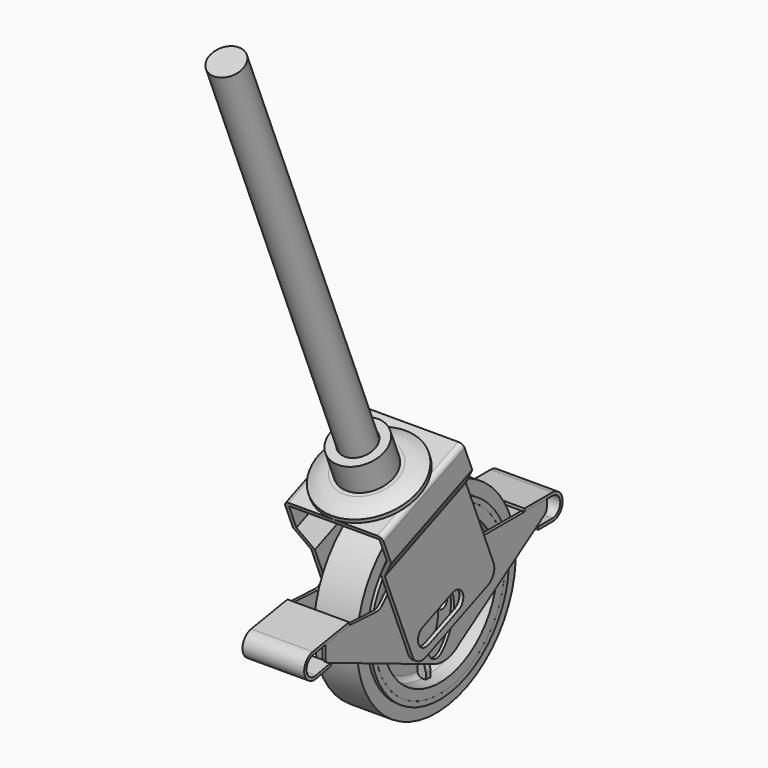
from build123d import *

# Parameters (mm, degrees)
F3_DEPTH  = 3
F4_R      = 5
F5_R      = 6
F6_DEPTH  = 55
F7_COUNT  = 6
F12_R     = 5
F13_DEPTH = 3
F16_DEPTH = 62
F18_DEPTH = 62
F21_DEPTH = 55
F22_R     = 13
F24_DEPTH = 4
F26_R     = 17.5
F27_DEPTH = 4
F30_R     = 17.5
F31_DEPTH = 10
F32_R     = 27
F32_R_2   = 17.5
F33_DEPTH = 30
F35_R     = 17
F36_DEPTH = 500


# Not quite as in the source:
# - ends of sketch curves that miss each other by under 0.0002 mm in the source are joined
# - a pattern or mirror of a feature is missing from the dataset's text; its kind, count and spacing are read off the source's solid


with BuildPart() as f1:
    # F0 (on Front) → F1 (revolve)
    with BuildSketch(Plane.XZ):
        Polygon((0, 82), (0, 0), (27.5, 0), (27.5, 22), (5, 22), (5, 72), (25, 72), (25, 82), align=None)
        Polygon((-27.5, 0), (0, 0), (0, 82), (-25, 82), (-25, 72), (-5, 72), (-5, 22), (-27.5, 22), align=None)
    revolve(axis=Axis((-13.75, 0, 0), (1, 0, 0)))

    # F4
    f4_edges = [f1.edges().sort_by_distance(p)[0] for p in [
        (5, 0, -72),
        (-5, 0, -72),
    ]]
    fillet(f4_edges, radius=F4_R)

    # F5 (on face) → F6 (cut, through all)
    with BuildSketch(Plane.YZ.offset(27.5)):
        Circle(F5_R)
    extrude(amount=-F6_DEPTH, mode=Mode.SUBTRACT)


with BuildPart() as f3:
    # F2 (on Front) → F3 (new body, symmetric)
    with BuildSketch(Plane.XZ):
        with BuildLine():
            ThreePointArc((10, 72), (6.4644660941, 70.5355339059), (5, 67))
            Line((5, 67), (5, 22))
            Line((5, 22), (13.5, 22))
            Line((13.5, 22), (11, 36.5))
            Line((11, 36.5), (11, 56.5))
            Line((11, 56.5), (13.5, 65.5393302441))
            Line((13.5, 65.5393302441), (13.5, 72))
            Line((13.5, 72), (10, 72))
        make_face()
    extrude(amount=F3_DEPTH, both=True)


with BuildPart() as f7_1:
    # F7: instance of F3
    add(f3.part.rotate(Axis((27.5, 0, 0), (1, 0, 0)), 1 * 360 / F7_COUNT))


with BuildPart() as f7_2:
    # F7: instance of F3
    add(f3.part.rotate(Axis((27.5, 0, 0), (1, 0, 0)), 2 * 360 / F7_COUNT))


with BuildPart() as f7_3:
    # F7: instance of F3
    add(f3.part.rotate(Axis((27.5, 0, 0), (1, 0, 0)), 3 * 360 / F7_COUNT))


with BuildPart() as f7_4:
    # F7: instance of F3
    add(f3.part.rotate(Axis((27.5, 0, 0), (1, 0, 0)), 4 * 360 / F7_COUNT))


with BuildPart() as f7_5:
    # F7: instance of F3
    add(f3.part.rotate(Axis((27.5, 0, 0), (1, 0, 0)), 5 * 360 / F7_COUNT))


with BuildPart() as f8_1:
    # F8: instance of F3
    add(f3.part.mirror(Plane.YZ))


with BuildPart() as f8_2:
    # F8: instance of F7_5
    add(f7_5.part.mirror(Plane.YZ))


with BuildPart() as f8_3:
    # F8: instance of F7_4
    add(f7_4.part.mirror(Plane.YZ))


with BuildPart() as f8_4:
    # F8: instance of F7_3
    add(f7_3.part.mirror(Plane.YZ))


with BuildPart() as f8_5:
    # F8: instance of F7_2
    add(f7_2.part.mirror(Plane.YZ))


with BuildPart() as f8_6:
    # F8: instance of F7_1
    add(f7_1.part.mirror(Plane.YZ))


with BuildPart() as f10:
    # F9 (on Top) → F10 (revolve)
    with BuildSketch(Plane.XY):
        Polygon((21.4822281301, -87), (25, -87), (25, -82), (-25, -82), (-25, -87), (-21.5177718699, -87), (-21.5177718699, -100), (21.4822281301, -100), align=None)
    revolve(axis=Axis((27.5, 0, 0), (-1, 0, 0)))


with BuildPart() as f13:
    # F12 (on offset) → F13 (new body)
    with BuildSketch(Plane.YZ.offset(28)):
        with BuildLine():
            Line((127, 41), (31.8588500737, 41))
            ThreePointArc((31.8588500737, 41), (26.284303624, 42.6979260495), (22.6027907005, 47.215113624))
            Line((22.6027907005, 47.215113624), (-3, 109.8275482655))
            Line((-3, 109.8275482655), (-27, 109.8275482655))
            Line((-27, 109.8275482655), (-34.8811647981, 80.414640816))
            ThreePointArc((-34.8811647981, 80.414640816), (-35.8106777129, 78.1251734114), (-37.2731987832, 76.1335189801))
            Line((-37.2731987832, 76.1335189801), (-79.5964464014, 31.3586536425))
            ThreePointArc((-79.5964464014, 31.3586536425), (-83.1487583061, 28.9436013276), (-87.3865234615, 28.2416440355))
            Line((-87.3865234615, 28.2416440355), (-120.9705632925, 30))
            Line((-120.9705632925, 30), (-150.9705632925, 25))
            Line((-150.9705632925, 25), (-150.9705632925, 12.3368176915))
            ThreePointArc((-150.9705632925, 12.3368176915), (-150.1294766363, 9.5613105669), (-147.8891873731, 7.7195802449))
            Line((-147.8891873731, 7.7195802449), (-14.5117444834, -47.7034246791))
            ThreePointArc((-14.5117444834, -47.7034246791), (1.9327525953, -49.5916872083), (16.8755716943, -42.4713517579))
            Line((16.8755716943, -42.4713517579), (124.7486402107, 28.5184114939))
            ThreePointArc((124.7486402107, 28.5184114939), (126.4013180443, 30.3227051329), (127, 32.6951299416))
            Line((127, 32.6951299416), (127, 41))
        make_face()
        with BuildLine():
            ThreePointArc((-9.9237075462, -1.2328943736), (-1.2328943736, 9.9237075462), (9.9237075462, 1.2328943736))
            ThreePointArc((9.9237075462, 1.2328943736), (7.4805498352, -21.4991216683), (-4.8262924538, -40.7671056264))
            ThreePointArc((-4.8262924538, -40.7671056264), (-18.9671056264, -40.5737075462), (-18.7737075462, -26.4328943736))
            ThreePointArc((-18.7737075462, -26.4328943736), (-11.3896021729, -14.8721039988), (-9.9237075462, -1.2328943736))
        make_face(mode=Mode.SUBTRACT)
        with Locations((-53.5, 36.5)):
            Circle(F12_R, mode=Mode.SUBTRACT)
    extrude(amount=F13_DEPTH)


with BuildPart() as f14_1:
    # F14: instance of F13
    add(f13.part.mirror(Plane.YZ))


with BuildPart() as f16:
    # F15 (on face) → F16 (new body, through all)
    with BuildSketch(Plane.YZ.offset(31)):
        with BuildLine():
            ThreePointArc((-163.0315809071, 2.71851264), (-174.8087468604, 10.7370416197), (-166.6145531656, 22.3926683545))
            Line((-166.6145531656, 22.3926683545), (-120.9705632925, 30))
            Line((-120.9705632925, 30), (-121.4637602544, 32.9591817715))
            Line((-121.4637602544, 32.9591817715), (-167.1077501275, 25.351850126))
            ThreePointArc((-167.1077501275, 25.351850126), (-177.7602019307, 10.1995353708), (-162.4498861915, -0.2245523028))
            Line((-162.4498861915, -0.2245523028), (-144.0324838866, 3.4156343068))
            Line((-144.0324838866, 3.4156343068), (-144.6141786022, 6.3586992496))
            Line((-144.6141786022, 6.3586992496), (-163.0315809071, 2.71851264))
        make_face()
    extrude(amount=-F16_DEPTH)


with BuildPart() as f18:
    # F17 (on face) → F18 (new body, through all)
    with BuildSketch(Plane.YZ.offset(31)):
        with BuildLine():
            Line((99, 41), (127, 41))
            Line((127, 41), (134, 41))
            ThreePointArc((134, 41), (143.9999581909, 30.9710832071), (133.942166656, 21.0001672362))
            Line((133.942166656, 21.0001672362), (116.2890405931, 21.0001672362))
            Line((116.2890405931, 21.0001672362), (116.2890405931, 18.0001672362))
            Line((116.2890405931, 18.0001672362), (133.9248166528, 18.0001672362))
            Line((133.9248166528, 18.0001672362), (133.942166656, 18.0001672362))
            ThreePointArc((133.942166656, 18.0001672362), (146.9999678391, 30.9710831706), (134, 44))
            Line((134, 44), (99, 44))
            Line((99, 44), (99, 41))
        make_face()
    extrude(amount=-F18_DEPTH)


with BuildPart() as f21:
    # F20 (on offset) → F21 (new body, symmetric)
    with BuildSketch(Plane(origin=(0, -0.0077183482, -0.0031561024), x_dir=(-1, 0, 0), z_dir=(0, 0.9256059373, 0.3784886376))):
        with BuildLine():
            Line((0, 133.5), (44.5, 133.5))
            ThreePointArc((44.5, 133.5), (45.2071067812, 133.2071067812), (45.5, 132.5))
            Line((45.5, 132.5), (45.5, 108.65))
            Line((45.5, 108.65), (33, 88.65))
            Line((33, 88.65), (33, -17.5))
            Line((33, -17.5), (37, -17.5))
            Line((37, -17.5), (37, 87.5028150944))
            Line((37, 87.5028150944), (49.5, 107.5028150944))
            Line((49.5, 107.5028150944), (49.5, 132.5))
            ThreePointArc((49.5, 132.5), (48.0355339059, 136.0355339059), (44.5, 137.5))
            Line((44.5, 137.5), (0, 137.5))
            Line((0, 137.5), (-44.5, 137.5))
            ThreePointArc((-44.5, 137.5), (-48.0355339059, 136.0355339059), (-49.5, 132.5))
            Line((-49.5, 132.5), (-49.5, 107.5028150944))
            Line((-49.5, 107.5028150944), (-37, 87.5028150944))
            Line((-37, 87.5028150944), (-37, -17.5))
            Line((-37, -17.5), (-33, -17.5))
            Line((-33, -17.5), (-33, 88.65))
            Line((-33, 88.65), (-45.5, 108.65))
            Line((-45.5, 108.65), (-45.5, 132.5))
            ThreePointArc((-45.5, 132.5), (-45.2071067812, 133.2071067812), (-44.5, 133.5))
            Line((-44.5, 133.5), (0, 133.5))
        make_face()
    extrude(amount=F21_DEPTH, both=True)

    # F22
    f22_edges = [f21.edges().sort_by_distance(p)[0] for p in [
        (35, 57.524159, 4.615615),
        (35, -44.292494, -37.018135),
        (-35, -44.292494, -37.018135),
        (-35, 57.524159, 4.615615),
    ]]
    fillet(f22_edges, radius=F22_R)

    # F23 (on face) → F24 (cut, through all)
    with BuildSketch(Plane(origin=(-37, 0, 0), x_dir=(0, -1, 0), z_dir=(-1, 0, 0))):
        with BuildLine():
            Line((-0.8930430629, 11.1687503692), (-0.7934201853, 11.1280140947))
            ThreePointArc((-0.7934201853, 11.1280140947), (-0.8431768183, 11.1485162628), (-0.8930430629, 11.1687503692))
        make_face()
        with BuildLine():
            Line((36.1810606746, -3.9910292413), (-0.7934201853, 11.1280140947))
            Line((-0.7934201853, 11.1280140947), (-0.8930430629, 11.1687503692))
            ThreePointArc((-0.8930430629, 11.1687503692), (-13.9403236987, 5.5367785502), (-8.1813671125, -7.4549518041))
            Line((-8.1813671125, -7.4549518041), (28.6106000979, -22.5028666972))
            ThreePointArc((28.6106000979, -22.5028666972), (41.6521265419, -17.0323326076), (36.1810606746, -3.9910292413))
        make_face()
    f24 = extrude(amount=-F24_DEPTH, mode=Mode.SUBTRACT)

    # F24_copies: F24 across plane
    add(f24.mirror(Plane(origin=(0, 0, 0), x_dir=(0, 0, 1), z_dir=(1, 0, 0))), mode=Mode.SUBTRACT)

    # F26 (on face) → F27 (cut, through all)
    with BuildSketch(Plane(origin=(0, -52.0421876702, 127.2708163818), x_dir=(1, 0, 0), z_dir=(0, -0.3784886376, 0.9256059373))):
        with Locations((0, -5.0083386979)):
            Circle(F26_R)
    extrude(amount=-F27_DEPTH, mode=Mode.SUBTRACT)


with BuildPart() as f29:
    # F28 (on offset) → F29 (revolve)
    with BuildSketch(Plane(origin=(0, 0, 0), x_dir=(0, -1, 0), z_dir=(-1, 0, 0))):
        with BuildLine():
            Line((60.4628220811, 134.6312764647), (56.6779357051, 125.3752170914))
            Line((56.6779357051, 125.3752170914), (102.9582325712, 106.4507852114))
            Line((102.9582325712, 106.4507852114), (104.4721871216, 110.1532089606))
            ThreePointArc((104.4721871216, 110.1532089606), (97.7586262502, 117.7219228943), (89.0836831737, 122.9279475586))
            Line((89.0836831737, 122.9279475586), (60.4628220811, 134.6312764647))
        make_face()
    revolve(axis=Axis((0, -58.5703788931, 130.003246778), (0, -0.3784886376, 0.9256059373)))

    # F30 (on face) → F31 (cut)
    with BuildSketch(Plane(origin=(0, -55.8270740462, 136.5268757551), x_dir=(1, 0, 0), z_dir=(0, -0.3784886376, 0.9256059373))):
        with Locations((0, -5.0083386979)):
            Circle(F30_R)
    extrude(amount=-F31_DEPTH, mode=Mode.SUBTRACT)

    # F32 (on face) → F33 (join)
    with BuildSketch(Plane(origin=(0, -55.8270740462, 136.5268757551), x_dir=(1, 0, 0), z_dir=(0, -0.3784886376, 0.9256059373))):
        with Locations((0, -5.0083386979)):
            Circle(F32_R)
        with Locations((0, -5.0083386979)):
            Circle(F32_R_2, mode=Mode.SUBTRACT)
    extrude(amount=F33_DEPTH)


with BuildPart() as f36:
    # F35 (on offset) → F36 (new body)
    with BuildSketch(Plane(origin=(0, -42.9584603678, 105.0562738861), x_dir=(1, 0, 0), z_dir=(0, 0.3784886376, -0.9256059373))):
        with Locations((0, 5.1940311678)):
            Circle(F35_R)
    extrude(amount=-F36_DEPTH)


solid = Compound([f1.part, f3.part, f7_1.part, f7_2.part, f7_3.part, f7_4.part, f7_5.part, f8_1.part, f8_2.part, f8_3.part, f8_4.part, f8_5.part, f8_6.part, f10.part, f13.part, f14_1.part, f16.part, f18.part, f21.part, f29.part, f36.part])
